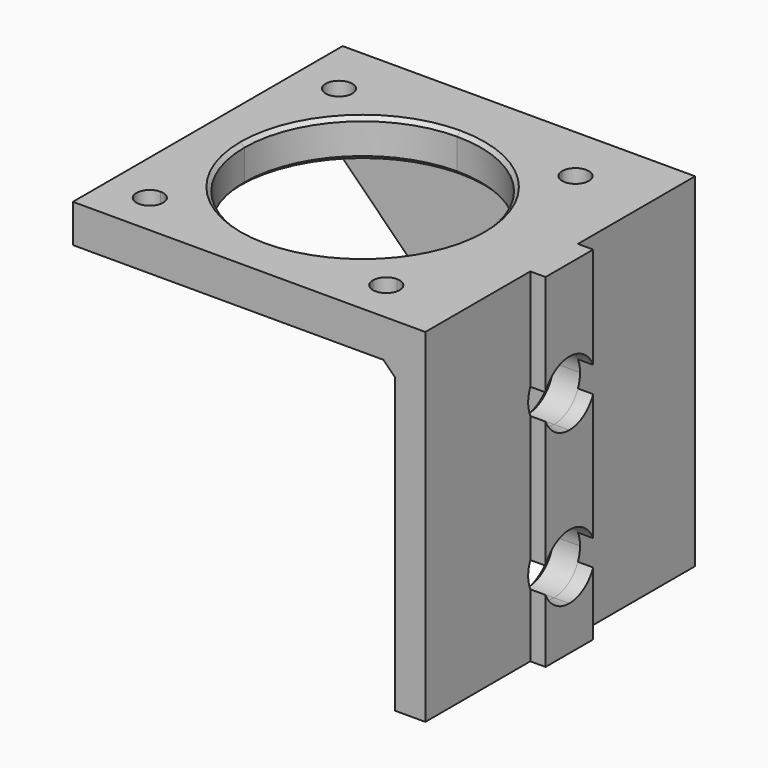
from build123d import *

# Parameters (mm, degrees)
F0_W      = 42.2
F0_H      = 42.2
F1_DEPTH  = 5
F2_DEPTH  = 40
F3_DEPTH  = 2
F5_DEPTH  = 25
F4_W      = 3.9
F4_H      = 6.5
F6_DEPTH  = 2
F7_SIZE   = 0.5
F8_SIZE   = 35
F9_DEPTH  = 16.75
F10_DEPTH = 21.75
F11_DEPTH = 25
F12_SIZE  = 1.5


# Not quite as in the source:
# - a feature names something its author has since deleted; it is built from what else it names


with BuildPart() as f1:
    # F0 (on Top) → F1 (new body)
    with BuildSketch(Plane.XY):
        Rectangle(F0_W, F0_H)
        with BuildLine():
            ThreePointArc((-15.5, 13.75), (-16.7374368671, 16.7374368671), (-13.75, 15.5))
            Line((-13.75, 15.5), (0, 15.5))
            Line((0, 15.5), (13.75, 15.5))
            ThreePointArc((13.75, 15.5), (15.5, 17.25), (17.25, 15.5))
            ThreePointArc((17.25, 15.5), (16.7374368671, 14.2625631329), (15.5, 13.75))
            Line((15.5, 13.75), (15.5, 0))
            Line((15.5, 0), (15.5, -13.75))
            ThreePointArc((15.5, -13.75), (16.7374368671, -14.2625631329), (17.25, -15.5))
            ThreePointArc((17.25, -15.5), (15.5, -17.25), (13.75, -15.5))
            Line((13.75, -15.5), (0, -15.5))
            Line((0, -15.5), (-13.75, -15.5))
            ThreePointArc((-13.75, -15.5), (-16.7374368671, -16.7374368671), (-15.5, -13.75))
            Line((-15.5, -13.75), (-15.5, 0))
            Line((-15.5, 0), (-15.5, 13.75))
        make_face(mode=Mode.SUBTRACT)
        Polygon((-21.1, 21.1), (21.1, 21.1), (21.1, -21.1), (23.1, -21.1), (23.1, 23.1), (-21.1, 23.1), align=None)
        with BuildLine():
            Line((0, 15.5), (-13.75, 15.5))
            ThreePointArc((-13.75, 15.5), (-14.2625631329, 14.2625631329), (-15.5, 13.75))
            Line((-15.5, 13.75), (-15.5, 0))
            ThreePointArc((-15.5, 0), (-10.9601551084, 10.9601551084), (0, 15.5))
        make_face()
        with BuildLine():
            ThreePointArc((0, -15.5), (-10.9601551084, -10.9601551084), (-15.5, 0))
            Line((-15.5, 0), (-15.5, -13.75))
            ThreePointArc((-15.5, -13.75), (-14.2625631329, -14.2625631329), (-13.75, -15.5))
            Line((-13.75, -15.5), (0, -15.5))
        make_face()
        with BuildLine():
            Line((15.5, -13.75), (15.5, 0))
            ThreePointArc((15.5, 0), (10.9601551084, -10.9601551084), (0, -15.5))
            Line((0, -15.5), (13.75, -15.5))
            ThreePointArc((13.75, -15.5), (14.2625631329, -14.2625631329), (15.5, -13.75))
        make_face()
        with BuildLine():
            Line((13.75, 15.5), (0, 15.5))
            ThreePointArc((0, 15.5), (10.9601551084, 10.9601551084), (15.5, 0))
            Line((15.5, 0), (15.5, 13.75))
            ThreePointArc((15.5, 13.75), (14.2625631329, 14.2625631329), (13.75, 15.5))
        make_face()
    extrude(amount=F1_DEPTH)

    # F0 (on Top) → F2 (join)
    with BuildSketch(Plane.XY):
        Polygon((-21.1, 21.1), (21.1, 21.1), (21.1, -21.1), (23.1, -21.1), (23.1, 23.1), (-21.1, 23.1), align=None)
    extrude(amount=-F2_DEPTH)

    # F3 (add): a face of the model
    f3_faces = [f1.faces().sort_by_distance(p)[0] for p in [
        (23.1, 1, -17.5),
    ]]
    extrude(f3_faces, amount=F3_DEPTH)

    # F4 (on face) → F5 (cut)
    with BuildSketch(Plane.YZ.offset(25.1)):
        with BuildLine():
            ThreePointArc((4.25, -10), (3.00520382, -6.99479618), (0, -5.75))
            Line((0, -5.75), (0, -10))
            Line((0, -10), (0, -14.25))
            ThreePointArc((0, -14.25), (3.00520382, -13.00520382), (4.25, -10))
        make_face()
        with BuildLine():
            Line((0, -10), (0, -5.75))
            ThreePointArc((0, -5.75), (-4.25, -10), (0, -14.25))
            Line((0, -14.25), (0, -10))
        make_face()
        with BuildLine():
            Line((0, -30), (0, -34.25))
            ThreePointArc((0, -34.25), (3.00520382, -33.00520382), (4.25, -30))
            Line((4.25, -30), (0, -30))
        make_face()
        with BuildLine():
            ThreePointArc((0, -25.75), (-4.25, -30), (0, -34.25))
            Line((0, -34.25), (0, -30))
            Line((0, -30), (0, -25.75))
        make_face()
        with BuildLine():
            ThreePointArc((4.25, -30), (3.00520382, -26.99479618), (0, -25.75))
            Line((0, -25.75), (0, -30))
            Line((0, -30), (4.25, -30))
        make_face()
    extrude(amount=-F5_DEPTH, mode=Mode.SUBTRACT)

    # F4 (on face) → F6 (join)
    with BuildSketch(Plane.YZ.offset(25.1)):
        with Locations((1.95, -20)):
            Rectangle(F4_W, F4_H)
        with Locations((-1.95, -20)):
            Rectangle(F4_W, F4_H)
    extrude(amount=F6_DEPTH)

    # F7
    f7_edges = [f1.edges().sort_by_distance(p)[0] for p in [
        (21.1, -4.25, -30),
        (21.1, -4.25, -10),
        (0, -15.5, 5),
        (0, -15.5, 0),
        (-17.25, 15.5, 0),
        (-15.5, -17.25, 0),
        (17.25, -15.5, 0),
        (15.5, 17.25, 0),
    ]]
    chamfer(f7_edges, length=F7_SIZE)

    # F8
    f8_edges = [f1.edges().sort_by_distance(p)[0] for p in [
        (-21.1, 22.1, -40),
    ]]
    chamfer(f8_edges, length=F8_SIZE)

    # F9 (add): a face of the model
    f9_faces = [f1.faces().sort_by_distance(p)[0] for p in [
        (26.1, 0, -23.25),
    ]]
    extrude(f9_faces, amount=F9_DEPTH)

    # F10 (add): a face of the model
    f10_faces = [f1.faces().sort_by_distance(p)[0] for p in [
        (26.1, 0, -16.75),
    ]]
    extrude(f10_faces, amount=F10_DEPTH)

    # F11 (cut): faces of the model
    f11_faces = [f1.faces().sort_by_distance(p)[0] for p in [
        (25.1, 0, -10),
        (25.1, 0, -30),
    ]]
    extrude(f11_faces, amount=-F11_DEPTH, mode=Mode.SUBTRACT)

    # F12
    f12_edges = [f1.edges().sort_by_distance(p)[0] for p in [
        (21.1, 0, 0),
        (21.1, 21.1, -20),
        (0, 21.1, 0),
    ]]
    chamfer(f12_edges, length=F12_SIZE)


solid = f1.part
